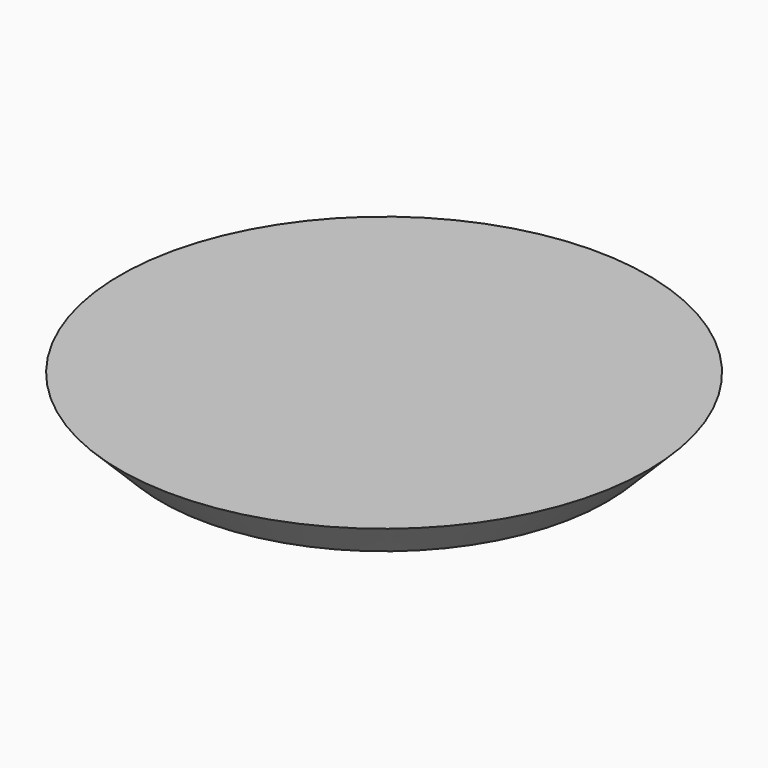
from build123d import *

# Parameters (mm, degrees)
F0_R     = 12.75
F1_DEPTH = 2
F2_SIZE  = 1.99999
F3_R     = 4
F4_DEPTH = 3.5


# Not quite as in the source:
# - a fillet or chamfer is up to 0.001 mm smaller than in the source, because OpenCascade refuses the exact size


with BuildPart() as f1:
    # F0 (on Top) → F1 (new body)
    with BuildSketch(Plane.XY):
        Circle(F0_R)
    extrude(amount=F1_DEPTH)

    # F2 (size 2 in the source; OpenCascade refuses exactly that, so slightly less here)
    f2_edges = [f1.edges().sort_by_distance(p)[0] for p in [
        (-12.75, 0, 0),
    ]]
    chamfer(f2_edges, length=F2_SIZE)

    # F3 (on face) → F4 (join)
    with BuildSketch(Plane(origin=(0, 0, 0), x_dir=(1, 0, 0), z_dir=(0, 0, -1))):
        Circle(F3_R)
    extrude(amount=F4_DEPTH)


solid = f1.part
